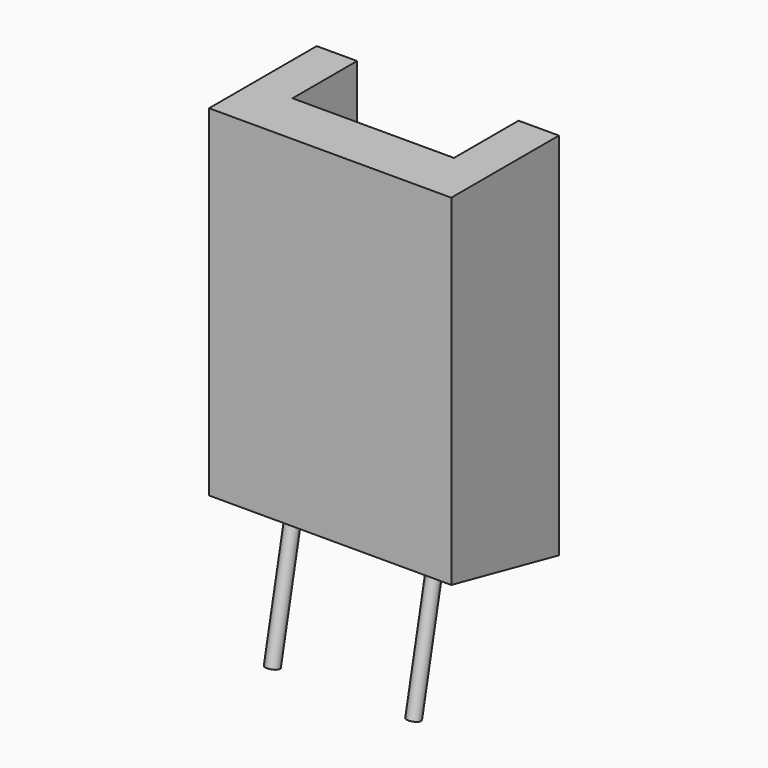
from build123d import *

# Parameters (mm, degrees)
F1_DEPTH      = 7.62
F1_DEPTH_BACK = 38.1
F2_DEPTH      = 15.24
F3_W          = 30.48
F3_H          = 15.24
F4_DEPTH      = 152.4
F5_R          = 1.27
F5_R_2        = 1.2522055882
F6_DEPTH      = 25.4


# Not quite as in the source:
# - a feature names something its author has since deleted; it is built from what else it names


with BuildPart() as f1:
    # F0 (on Right) → F1 (new body, two sides)
    with BuildSketch(Plane.YZ) as f1_sk:
        Polygon((-19.9023338153, 49.1049804437), (-37.6823338153, 49.1049804437), (-37.6823338153, -16.8750494665), (-19.9023338153, -20.654305133), align=None)
        Polygon((-37.6823338153, 49.1049804437), (-45.3023338153, 49.1049804437), (-45.3023338153, -15.2553684666), (-37.6823338153, -16.8750494665), align=None)
    extrude(amount=F1_DEPTH)
    extrude(f1_sk.sketch, amount=-F1_DEPTH_BACK)

    # F0 (on Right) → F2 (join)
    with BuildSketch(Plane.YZ):
        Polygon((-37.6823338153, 49.1049804437), (-45.3023338153, 49.1049804437), (-45.3023338153, -15.2553684666), (-37.6823338153, -16.8750494665), align=None)
    extrude(amount=-F2_DEPTH)

    # F3 (on face) → F4 (cut)
    with BuildSketch(Plane.XY.offset(49.1049804437)):
        with Locations((-15.24, -27.5223338153)):
            Rectangle(F3_W, F3_H)
    extrude(amount=-F4_DEPTH, mode=Mode.SUBTRACT)

    # F5 (on face) → F6 (join)
    with BuildSketch(Plane(origin=(0, -5.0607549484, -23.8089801067), x_dir=(1, 0, 0), z_dir=(0, -0.2079116908, -0.9781476007))):
        with Locations((-28.575, 32.6586192333)):
            Circle(F5_R)
        with Locations((-1.905, 32.6586192333)):
            Circle(F5_R_2)
    extrude(amount=F6_DEPTH)


solid = f1.part
